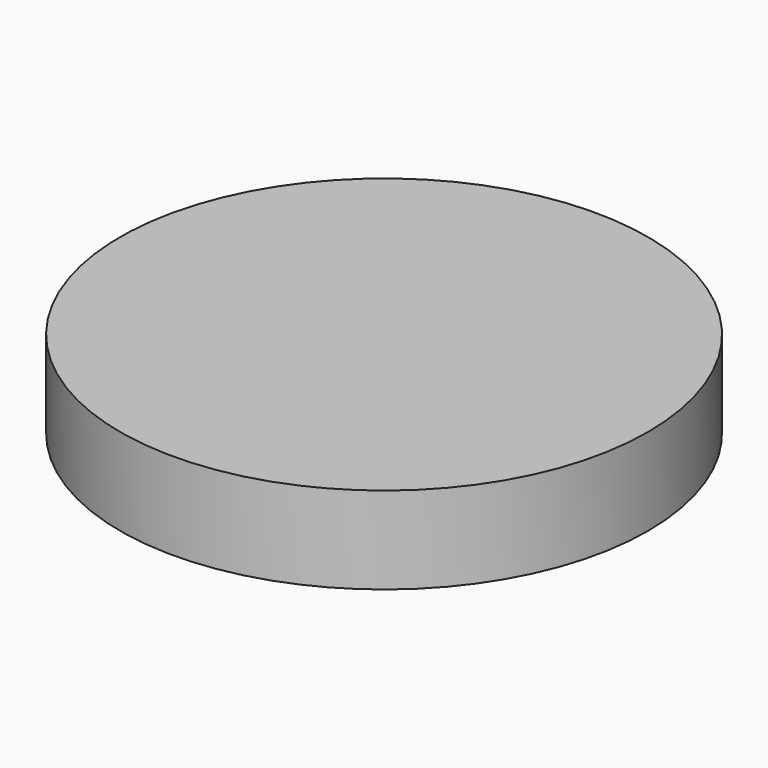
from build123d import *

# Parameters (mm, degrees)
F0_R     = 75.7666351468
F1_DEPTH = 25


# Not quite as in the source:
# - a feature names something its author has since deleted; it is built from what else it names


with BuildPart() as f1:
    # F0 (on Top) → F1 (new body)
    with BuildSketch(Plane.XY):
        with Locations((-6.0433540493, -23.9433422685)):
            Circle(F0_R)
    extrude(amount=F1_DEPTH)


solid = f1.part
